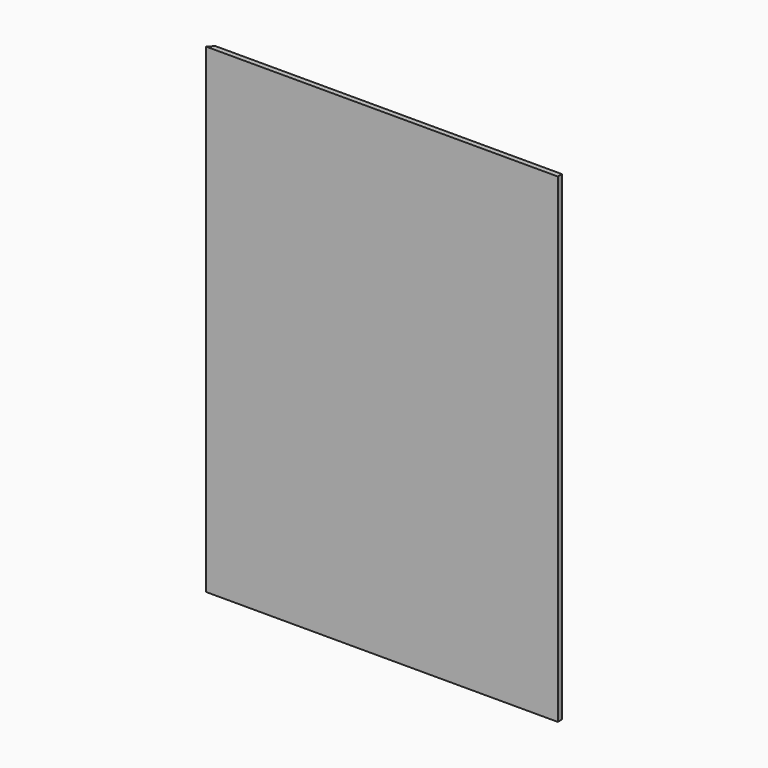
from build123d import *

# Parameters (mm, degrees)
F0_W        = 215.9
F0_H        = 292.1
F1_DEPTH    = 1.5875
F2_T1_DEPTH = 318.2282991577


# Not quite as in the source:
# - a fillet or chamfer that OpenCascade refuses, or shapes differently, is made with other operations: its cross-section is extruded or revolved along the edge and cut away or added


with BuildPart() as f1:
    # F0 (on Front) → F1 (new body, symmetric)
    with BuildSketch(Plane.XZ):
        Rectangle(F0_W, F0_H)
    extrude(amount=F1_DEPTH, both=True)

    # F2: chamfer of 5.08 on 1 edges, made by hand

    # F2_s2 → F2_t1 (cut)
    with BuildSketch(Plane.XY.offset(-159.1141495789)):
        Polygon((-107.95, -3.4925), (-102.87, 1.5875), (-107.95, 1.5875), align=None)
    extrude(amount=F2_T1_DEPTH, mode=Mode.SUBTRACT)


solid = f1.part
